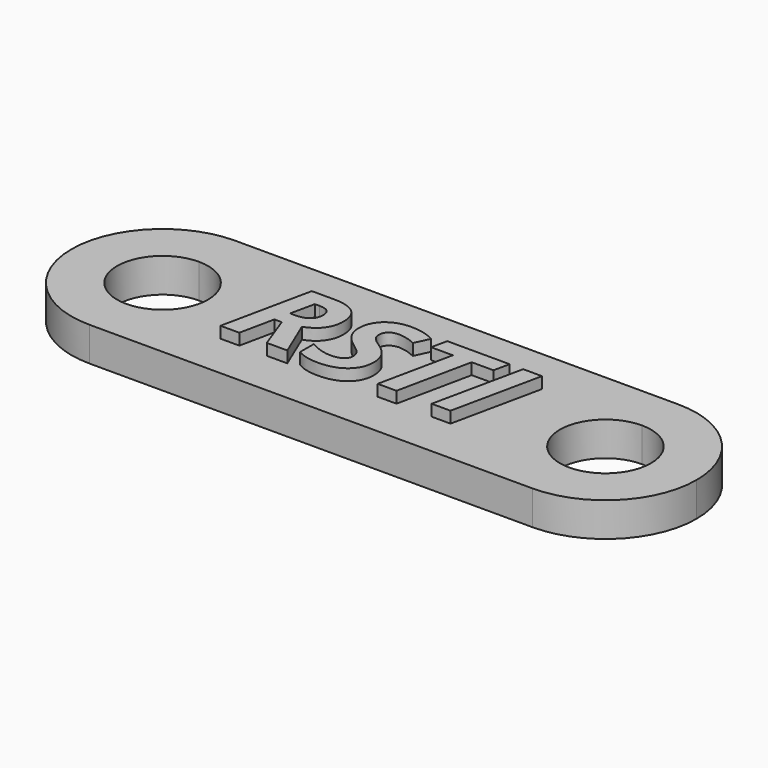
from build123d import *

# Parameters (mm, degrees)
F3_DEPTH     = 3
F1_TEXT_SIZE = 11.1111111111
F4_DEPTH     = 2
F5_DEPTH     = 3


# Not quite as in the source:
# - Text() gives the source's letters only with a copy of the font that has no kerning and outlines rounded to 1/6400 em; it was checked with that copy


with BuildPart() as f3:
    # F2 (on Top) → F3 (new body)
    with BuildSketch(Plane.XY):
        with BuildLine():
            ThreePointArc((-8, -4), (-2.3431457505, -1.6568542495), (0, 4))
            ThreePointArc((0, 4), (-2.3431457505, 9.6568542495), (-8, 12))
            Line((-8, 12), (-8, 8))
            ThreePointArc((-8, 8), (-5.1715728753, 6.8284271247), (-4, 4))
            ThreePointArc((-4, 4), (-5.1715728753, 1.1715728753), (-8, 0))
            Line((-8, 0), (-8, -4))
        make_face()
        with BuildLine():
            ThreePointArc((-8, 12), (-2.3431457505, 9.6568542495), (0, 4))
            ThreePointArc((0, 4), (-2.3431457505, -1.6568542495), (-8, -4))
            Line((-8, -4), (30.90625, -4))
            ThreePointArc((30.90625, -4), (22.90625, 4), (30.90625, 12))
            Line((30.90625, 12), (-8, 12))
        make_face()
        with BuildLine():
            Line((-8, 8), (-8, 12))
            ThreePointArc((-8, 12), (-16, 4), (-8, -4))
            Line((-8, -4), (-8, 0))
            ThreePointArc((-8, 0), (-12, 4), (-8, 8))
        make_face()
        with BuildLine():
            Line((30.90625, 8), (30.90625, 12))
            ThreePointArc((30.90625, 12), (22.90625, 4), (30.90625, -4))
            Line((30.90625, -4), (30.90625, 0))
            ThreePointArc((30.90625, 0), (26.90625, 4), (30.90625, 8))
        make_face()
        with BuildLine():
            ThreePointArc((38.90625, 4), (36.5631042495, 9.6568542495), (30.90625, 12))
            Line((30.90625, 12), (30.90625, 8))
            ThreePointArc((30.90625, 8), (33.7346771247, 6.8284271247), (34.90625, 4))
            ThreePointArc((34.90625, 4), (33.7346771247, 1.1715728753), (30.90625, 0))
            Line((30.90625, 0), (30.90625, -4))
            ThreePointArc((30.90625, -4), (36.5631042495, -1.6568542495), (38.90625, 4))
        make_face()
    extrude(amount=F3_DEPTH)

    # F1 (on offset) → F4 (cut, through all)
    with BuildSketch(Plane.XY.offset(1)):
        with Locations((0, 0)):
            Text('RSTI', F1_TEXT_SIZE, font='Open Sans', font_style=FontStyle.BOLDITALIC, text_align=(TextAlign.LEFT, TextAlign.BOTTOM))
    extrude(amount=F4_DEPTH, mode=Mode.SUBTRACT)


with BuildPart() as f5:
    # F1 (on offset) → F5 (new body)
    with BuildSketch(Plane.XY.offset(1)):
        with Locations((0, 0)):
            Text('RSTI', F1_TEXT_SIZE, font='Open Sans', font_style=FontStyle.BOLDITALIC, text_align=(TextAlign.LEFT, TextAlign.BOTTOM))
    extrude(amount=F5_DEPTH)


solid = Compound([f3.part, f5.part])
